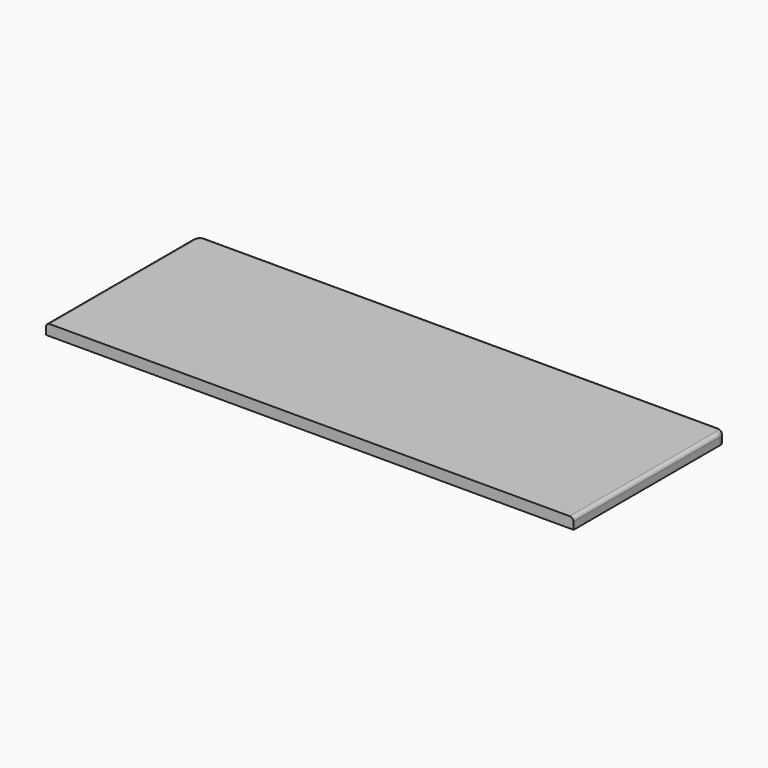
from build123d import *

# Parameters (mm, degrees)
F1_DEPTH    = 914.4
F2_R        = 6.35
F3_T1_DEPTH = 50.8
F3_T4_ANGLE = 90
F3_T6_ANGLE = 90


# Not quite as in the source:
# - a fillet or chamfer that OpenCascade refuses, or shapes differently, is made with other operations: its cross-section is extruded or revolved along the edge and cut away or added


with BuildPart() as f1:
    # F0 (on Right) → F1 (new body)
    with BuildSketch(Plane.YZ):
        Polygon((183.430065248, -26.0955506578), (-146.769934752, -26.0955506578), (-146.2517950619, -45.1455506578), (183.430065248, -45.1455506578), align=None)
    extrude(amount=F1_DEPTH)

    # F2
    f2_edges = [f1.edges().sort_by_distance(p)[0] for p in [
        (0, 18.330065, -26.095551),
        (457.2, 183.430065, -26.095551),
        (914.4, 18.330065, -26.095551),
    ]]
    fillet(f2_edges, radius=F2_R)

    # F3: fillet of radius 12.7 on 2 edges, made by hand

    # F3_s2 → F3_t1 (cut)
    with BuildSketch(Plane.XY.offset(-76.8955506578)):
        with BuildLine():
            ThreePointArc((914.4, 170.730065248), (910.6802561211, 179.710321369), (901.7, 183.430065248))
            Line((901.7, 183.430065248), (914.4, 183.430065248))
            Line((914.4, 183.430065248), (914.4, 170.730065248))
        make_face()
        with BuildLine():
            ThreePointArc((0, 170.730065248), (3.7197438789, 179.710321369), (12.7, 183.430065248))
            Line((12.7, 183.430065248), (0, 183.430065248))
            Line((0, 183.430065248), (0, 170.730065248))
        make_face()
    extrude(amount=F3_T1_DEPTH, mode=Mode.SUBTRACT)

    # F3_s3 → F3_t4 (revolve, cut)
    with BuildSketch(Plane.YZ.offset(12.7)):
        with BuildLine():
            ThreePointArc((177.080065248, -26.0955506578), (181.5701933085, -27.9554225973), (183.430065248, -32.4455506578))
            Line((183.430065248, -32.4455506578), (183.430065248, -26.0955506578))
            Line((183.430065248, -26.0955506578), (177.080065248, -26.0955506578))
        make_face()
    revolve(axis=Axis((12.7, 170.730065248, -26.0955506578), (0, 0, 1)), revolution_arc=F3_T4_ANGLE, mode=Mode.SUBTRACT)

    # F3_s5 → F3_t6 (revolve, cut)
    with BuildSketch(Plane.XZ.offset(-170.730065248)):
        with BuildLine():
            ThreePointArc((908.05, -26.0955506578), (912.5401280605, -27.9554225973), (914.4, -32.4455506578))
            Line((914.4, -32.4455506578), (914.4, -26.0955506578))
            Line((914.4, -26.0955506578), (908.05, -26.0955506578))
        make_face()
    revolve(axis=Axis((901.7, 170.730065248, -26.0955506578), (0, 0, 1)), revolution_arc=F3_T6_ANGLE, mode=Mode.SUBTRACT)


solid = f1.part
